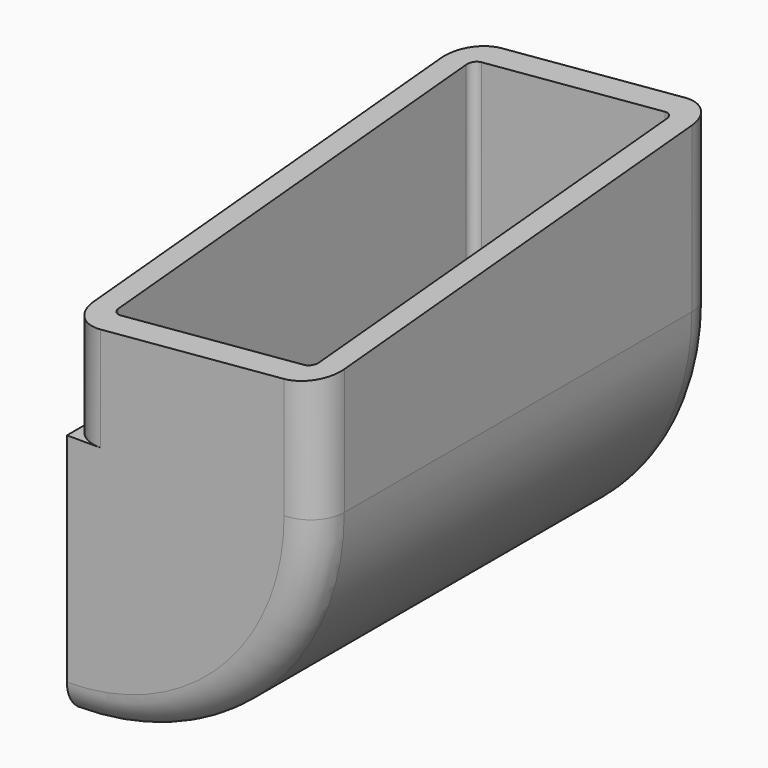
from build123d import *

# Parameters (mm, degrees)
F1_DEPTH  = 30
F2_T      = -3
F4_R      = 4
F6_DEPTH  = 20
F8_DEPTH  = 40
F11_DEPTH = 100
F13_R     = 1
F15_DEPTH = 25


# Not quite as in the source:
# - a feature of the source that left no trace in its solid (it failed there, or was rolled back) is left out


with BuildPart() as f1:
    # F0 (on Front) → F1 (new body, symmetric)
    with BuildSketch(Plane.XZ):
        with BuildLine():
            Line((0, 0), (0, -30))
            ThreePointArc((0, -30), (21.2132034356, -21.2132034356), (30, 0))
            Line((30, 0), (0, 0))
        make_face()
    extrude(amount=F1_DEPTH, both=True)

    # F2
    f2_openings = [f1.faces().sort_by_distance(p)[0] for p in [
        (15, 0, 0),
    ]]
    offset(amount=F2_T, openings=f2_openings)

    # F4
    f4_edges = [f1.edges().sort_by_distance(p)[0] for p in [
        (21.213203, -30, -21.213203),
        (21.213203, 30, -21.213203),
    ]]
    fillet(f4_edges, radius=F4_R)

    # F5 (on face) → F6 (join)
    with BuildSketch(Plane.XY):
        with BuildLine():
            Line((0, -30), (26, -30))
            ThreePointArc((26, -30), (28.8284271247, -28.8284271247), (30, -26))
            Line((30, -26), (30, 26))
            ThreePointArc((30, 26), (28.8284271247, 28.8284271247), (26, 30))
            Line((26, 30), (0, 30))
            Line((0, 30), (0, -30))
        make_face()
        Polygon((27, 26), (27, -26), (27, -27), (26, -27), (3, -27), (3, 27), (26, 27), (27, 27), align=None, mode=Mode.SUBTRACT)
    extrude(amount=F6_DEPTH)

    # F7 (on face) → F8 (cut)
    with BuildSketch(Plane(origin=(0, 0, 0), x_dir=(0, -1, 0), z_dir=(-1, 0, 0))):
        Polygon((30, 14.7506801884), (30, 20), (-30, 20), align=None)
    extrude(amount=-F8_DEPTH, mode=Mode.SUBTRACT)

    # F10 (on face) → F11 (cut)
    with BuildSketch(Plane(origin=(0, 31.5085980719, 2.7566451349), x_dir=(1, 0, 0), z_dir=(0, -0.9961946981, -0.0871557427))):
        Polygon((0, 14.6845617736), (30, 17.3092216794), (26, 17.3092216794), (0, 17.3092216794), align=None)
    extrude(amount=F11_DEPTH, mode=Mode.SUBTRACT)

    # F13
    f13_edges = [f1.edges().sort_by_distance(p)[0] for p in [
        (3, 27, -4.733249),
        (20.124612, 27, -18),
        (27, 27, 9.737033),
        (3, 0, -26.832816),
        (3, -27, -7.095443),
        (27, -27, 7.374839),
        (20.124612, -27, -18),
    ]]
    fillet(f13_edges, radius=F13_R)

    # F14 (on offset) → F15 (cut)
    with BuildSketch(Plane.XY.offset(25)):
        with BuildLine():
            Line((4, 30), (0, 30))
            Line((0, 30), (0, 26))
            ThreePointArc((0, 26), (1.1715728753, 28.8284271247), (4, 30))
        make_face()
        with BuildLine():
            Line((0, -26), (0, -30))
            Line((0, -30), (4, -30))
            ThreePointArc((4, -30), (1.1715728753, -28.8284271247), (0, -26))
        make_face()
    extrude(amount=-F15_DEPTH, mode=Mode.SUBTRACT)


solid = f1.part
